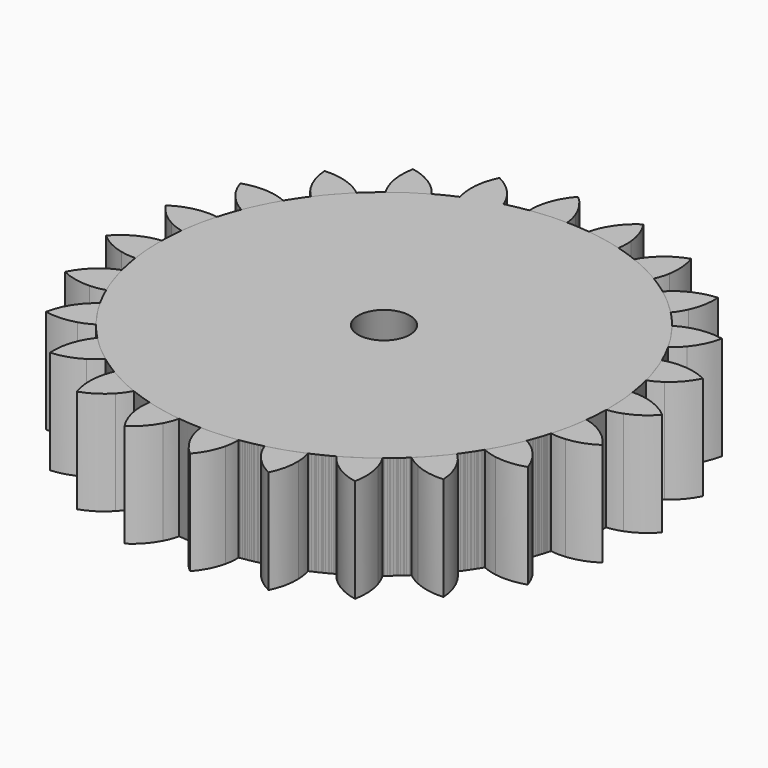
from build123d import *

# Parameters (mm, degrees)
F0_R     = 6.35
F1_DEPTH = 25.4
F2_COUNT = 24


# Not quite as in the source:
# - a feature of the source that left no trace in its solid (it failed there, or was rolled back) is left out


with BuildPart() as f1:
    # F0 (on Top) → F1 (new body)
    with BuildSketch(Plane.XY):
        with BuildLine():
            ThreePointArc((-7.8842675869, 53.139290225), (-35.0884247435, -40.6785974441), (53.721, 0))
            ThreePointArc((53.721, 0), (38.2966086664, 37.6738052983), (0.8807473744, 53.7137796572))
            ThreePointArc((0.8807473744, 53.7137796572), (-3.5135215054, 53.6059792153), (-7.8842675869, 53.139290225))
        make_face()
        Circle(F0_R, mode=Mode.SUBTRACT)
        with BuildLine():
            ThreePointArc((-8.0057647826, 54.5512037332), (-3.6060358558, 55.017475441), (0.8169134507, 55.129472616))
            ThreePointArc((0.8169134507, 55.129472616), (0.524413398, 56.928461046), (0, 58.674))
            ThreePointArc((0, 58.674), (-1.7395294034, 61.9989434499), (-4.2466275619, 64.791016213))
            ThreePointArc((-4.2466275619, 64.791016213), (-6.3678385219, 61.6955880433), (-7.6584938023, 58.1720357962))
            ThreePointArc((-7.6584938023, 58.1720357962), (-7.950582218, 56.3729804859), (-8.0057647826, 54.5512037332))
        make_face()
        with BuildLine():
            ThreePointArc((-7.8842675869, 53.139290225), (-3.5135215054, 53.6059792153), (0.8807473744, 53.7137796572))
            ThreePointArc((0.8807473744, 53.7137796572), (0.8668085526, 54.4224367751), (0.8169134507, 55.129472616))
            ThreePointArc((0.8169134507, 55.129472616), (-3.6060358558, 55.017475441), (-8.0057647826, 54.5512037332))
            ThreePointArc((-8.0057647826, 54.5512037332), (-7.9629463288, 53.8437040643), (-7.8842675869, 53.139290225))
        make_face()
        with BuildLine():
            ThreePointArc((0.8807473744, 53.7137796572), (38.2966086664, 37.6738052983), (53.721, 0))
            ThreePointArc((53.721, 0), (-35.0884247435, -40.6785974441), (-7.8842675869, 53.139290225))
            ThreePointArc((-7.8842675869, 53.139290225), (-7.9629463288, 53.8437040643), (-8.0057647826, 54.5512037332))
            ThreePointArc((-8.0057647826, 54.5512037332), (-36.0452774683, -41.7212664086), (55.135524832, 0))
            ThreePointArc((55.135524832, 0), (39.2744640342, 38.6968031409), (0.8169134507, 55.129472616))
            ThreePointArc((0.8169134507, 55.129472616), (0.8668085526, 54.4224367751), (0.8807473744, 53.7137796572))
        make_face()
    extrude(amount=F1_DEPTH)


with BuildPart() as f2_1:
    # F2: instance of F1
    add(f1.part.rotate(Axis((0, 0, 0), (0, 0, -1)), 1 * 360 / F2_COUNT))


with BuildPart() as f2_2:
    # F2: instance of F1
    add(f1.part.rotate(Axis((0, 0, 0), (0, 0, -1)), 2 * 360 / F2_COUNT))


with BuildPart() as f2_3:
    # F2: instance of F1
    add(f1.part.rotate(Axis((0, 0, 0), (0, 0, -1)), 3 * 360 / F2_COUNT))


with BuildPart() as f2_4:
    # F2: instance of F1
    add(f1.part.rotate(Axis((0, 0, 0), (0, 0, -1)), 4 * 360 / F2_COUNT))


with BuildPart() as f2_5:
    # F2: instance of F1
    add(f1.part.rotate(Axis((0, 0, 0), (0, 0, -1)), 5 * 360 / F2_COUNT))


with BuildPart() as f2_6:
    # F2: instance of F1
    add(f1.part.rotate(Axis((0, 0, 0), (0, 0, -1)), 6 * 360 / F2_COUNT))


with BuildPart() as f2_7:
    # F2: instance of F1
    add(f1.part.rotate(Axis((0, 0, 0), (0, 0, -1)), 7 * 360 / F2_COUNT))


with BuildPart() as f2_8:
    # F2: instance of F1
    add(f1.part.rotate(Axis((0, 0, 0), (0, 0, -1)), 8 * 360 / F2_COUNT))


with BuildPart() as f2_9:
    # F2: instance of F1
    add(f1.part.rotate(Axis((0, 0, 0), (0, 0, -1)), 9 * 360 / F2_COUNT))


with BuildPart() as f2_10:
    # F2: instance of F1
    add(f1.part.rotate(Axis((0, 0, 0), (0, 0, -1)), 10 * 360 / F2_COUNT))


with BuildPart() as f2_11:
    # F2: instance of F1
    add(f1.part.rotate(Axis((0, 0, 0), (0, 0, -1)), 11 * 360 / F2_COUNT))


with BuildPart() as f2_12:
    # F2: instance of F1
    add(f1.part.rotate(Axis((0, 0, 0), (0, 0, -1)), 12 * 360 / F2_COUNT))


with BuildPart() as f2_13:
    # F2: instance of F1
    add(f1.part.rotate(Axis((0, 0, 0), (0, 0, -1)), 13 * 360 / F2_COUNT))


with BuildPart() as f2_14:
    # F2: instance of F1
    add(f1.part.rotate(Axis((0, 0, 0), (0, 0, -1)), 14 * 360 / F2_COUNT))


with BuildPart() as f2_15:
    # F2: instance of F1
    add(f1.part.rotate(Axis((0, 0, 0), (0, 0, -1)), 15 * 360 / F2_COUNT))


with BuildPart() as f2_16:
    # F2: instance of F1
    add(f1.part.rotate(Axis((0, 0, 0), (0, 0, -1)), 16 * 360 / F2_COUNT))


with BuildPart() as f2_17:
    # F2: instance of F1
    add(f1.part.rotate(Axis((0, 0, 0), (0, 0, -1)), 17 * 360 / F2_COUNT))


with BuildPart() as f2_18:
    # F2: instance of F1
    add(f1.part.rotate(Axis((0, 0, 0), (0, 0, -1)), 18 * 360 / F2_COUNT))


with BuildPart() as f2_19:
    # F2: instance of F1
    add(f1.part.rotate(Axis((0, 0, 0), (0, 0, -1)), 19 * 360 / F2_COUNT))


with BuildPart() as f2_20:
    # F2: instance of F1
    add(f1.part.rotate(Axis((0, 0, 0), (0, 0, -1)), 20 * 360 / F2_COUNT))


with BuildPart() as f2_21:
    # F2: instance of F1
    add(f1.part.rotate(Axis((0, 0, 0), (0, 0, -1)), 21 * 360 / F2_COUNT))


with BuildPart() as f2_22:
    # F2: instance of F1
    add(f1.part.rotate(Axis((0, 0, 0), (0, 0, -1)), 22 * 360 / F2_COUNT))


with BuildPart() as f2_23:
    # F2: instance of F1
    add(f1.part.rotate(Axis((0, 0, 0), (0, 0, -1)), 23 * 360 / F2_COUNT))


solid = Compound([f1.part, f2_1.part, f2_2.part, f2_3.part, f2_4.part, f2_5.part, f2_6.part, f2_7.part, f2_8.part, f2_9.part, f2_10.part, f2_11.part, f2_12.part, f2_13.part, f2_14.part, f2_15.part, f2_16.part, f2_17.part, f2_18.part, f2_19.part, f2_20.part, f2_21.part, f2_22.part, f2_23.part])
